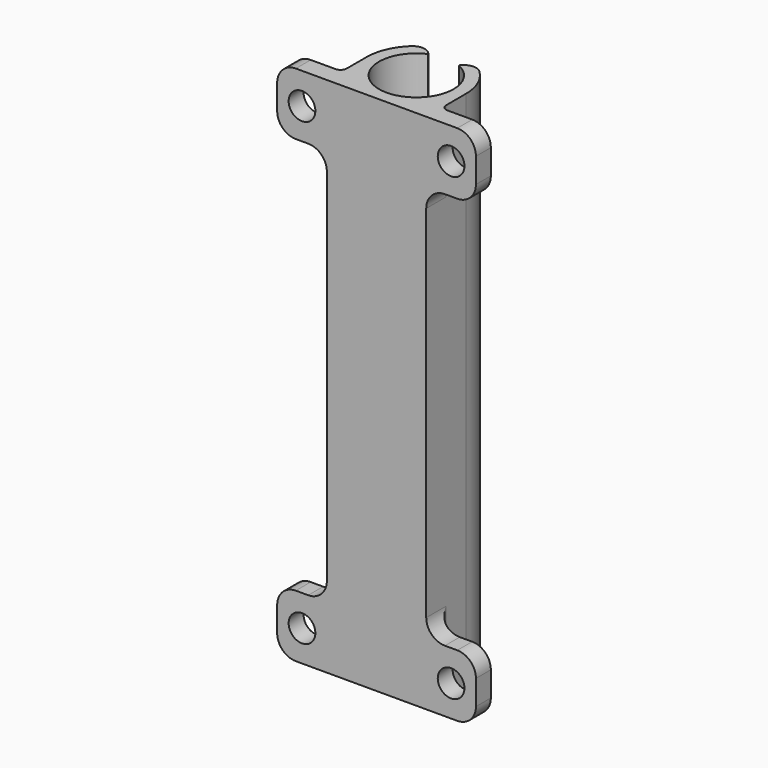
from build123d import *

# Parameters (mm, degrees)
F0_W        = 8
F0_H        = 3
F1_DEPTH    = 84
F3_D        = 4.3
F3_DEPTH    = 16
F3_START    = 5
F3_TIP      = 1.2918503309
F2_W        = 8
F2_H        = 64
F4_DEPTH    = 25
F5_R        = 3
F6_R        = 1
F7_T1_DEPTH = 101.4328702047


# Not quite as in the source:
# - a fillet or chamfer that OpenCascade refuses, or shapes differently, is made with other operations: its cross-section is extruded or revolved along the edge and cut away or added


with BuildPart() as f1:
    # F0 (on Top) → F1 (new body)
    with BuildSketch(Plane.XY):
        with Locations((-12, -6.5)):
            Rectangle(F0_W, F0_H)
        with BuildLine():
            ThreePointArc((0, -8), (-5.6568542495, -5.6568542495), (-8, 0))
            Line((-8, 0), (-8, -5))
            Line((-8, -5), (-8, -8))
            Line((-8, -8), (-2.5, -8))
            Line((-2.5, -8), (0, -8))
        make_face()
        with BuildLine():
            ThreePointArc((2.4590163934, 5.4729551777), (0, -6), (-2.4590163934, 5.4729551777))
            Line((-2.4590163934, 5.4729551777), (-2.5, 7.5993420768))
            ThreePointArc((-2.5, 7.5993420768), (-6.4807406984, 4.6904157598), (-8, 0))
            ThreePointArc((-8, 0), (-5.6568542495, -5.6568542495), (0, -8))
            ThreePointArc((0, -8), (5.6568542495, -5.6568542495), (8, 0))
            ThreePointArc((8, 0), (6.4807406984, 4.6904157598), (2.5, 7.5993420768))
            Line((2.5, 7.5993420768), (2.4590163934, 5.4729551777))
        make_face()
        with BuildLine():
            Line((8, -5), (8, 0))
            ThreePointArc((8, 0), (5.6568542495, -5.6568542495), (0, -8))
            Line((0, -8), (2.5, -8))
            Line((2.5, -8), (8, -8))
            Line((8, -8), (8, -5))
        make_face()
        with Locations((12, -6.5)):
            Rectangle(F0_W, F0_H)
    extrude(amount=F1_DEPTH)

    # F3
    # its depths count from where the whole tool has entered the part; down to there all is cleared
    with Locations(Plane(origin=(0, 0, 0), x_dir=(1, 0, 0), z_dir=(0, 1, 0)).offset(-F3_START)):
        with Locations((12, -5), (-12, -5), (12, -79), (-12, -79)):
            Hole(F3_D / 2, depth=F3_DEPTH)
            with Locations((0, 0, -(F3_DEPTH + F3_TIP / 2))):  # 118° drill point
                Cone(0, F3_D / 2, F3_TIP, mode=Mode.SUBTRACT)

    # F2 (on Front) → F4 (cut)
    with BuildSketch(Plane.XZ):
        with Locations((12, 42)):
            Rectangle(F2_W, F2_H)
        with Locations((-12, 42)):
            Rectangle(F2_W, F2_H)
    extrude(amount=F4_DEPTH, mode=Mode.SUBTRACT)

    # F5
    f5_edges = [f1.edges().sort_by_distance(p)[0] for p in [
        (-16, -6.5, 84),
        (-16, -6.5, 74),
        (16, -6.5, 84),
        (16, -6.5, 74),
        (-16, -6.5, 0),
        (16, -6.5, 0),
        (16, -6.5, 10),
        (-16, -6.5, 10),
        (-8, -6.5, 10),
        (8, -6.5, 10),
        (-8, -6.5, 74),
        (8, -6.5, 74),
    ]]
    fillet(f5_edges, radius=F5_R)

    # F6
    f6_edges = [f1.edges().sort_by_distance(p)[0] for p in [
        (-8, -5, 5),
        (8, -5, 5),
        (8, -5, 79),
        (-8, -5, 79),
    ]]
    fillet(f6_edges, radius=F6_R)

    # F7: fillet of radius 2 on 2 edges, made by hand

    # F7_s2 → F7_t1 (cut)
    with BuildSketch(Plane.XY.offset(-8.7164351024)):
        with BuildLine():
            ThreePointArc((2.4590163934, 5.4729551777), (3.8977705539, 6.3481743906), (5.4949420866, 5.8142593221))
            ThreePointArc((5.4949420866, 5.8142593221), (4.0959009817, 6.8719426036), (2.5, 7.5993420768))
            Line((2.5, 7.5993420768), (2.4590163934, 5.4729551777))
        make_face()
        with BuildLine():
            ThreePointArc((-5.4949420866, 5.8142593221), (-3.8977705539, 6.3481743906), (-2.4590163934, 5.4729551777))
            Line((-2.4590163934, 5.4729551777), (-2.5, 7.5993420768))
            ThreePointArc((-2.5, 7.5993420768), (-4.0959009817, 6.8719426036), (-5.4949420866, 5.8142593221))
        make_face()
    extrude(amount=F7_T1_DEPTH, mode=Mode.SUBTRACT)


solid = f1.part
